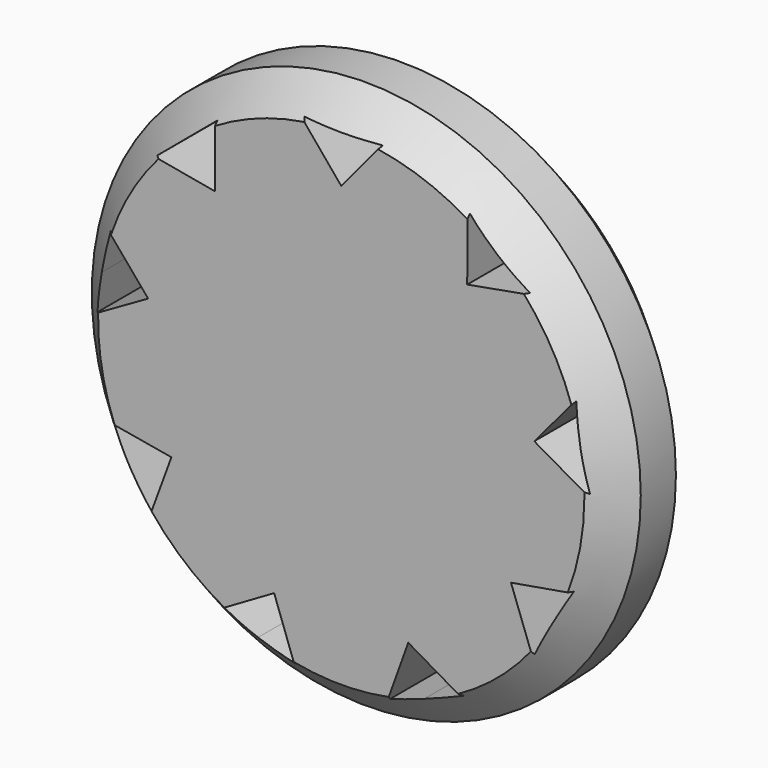
from build123d import *

# Parameters (mm, degrees)
F0_R     = 44.45
F1_DEPTH = 17.272
F3_DEPTH = 17.273


# Not quite as in the source:
# - a fillet or chamfer that OpenCascade refuses, or shapes differently, is made with other operations: its cross-section is extruded or revolved along the edge and cut away or added


with BuildPart() as f1:
    # F0 (on Front) → F1 (new body)
    with BuildSketch(Plane.XZ):
        Circle(F0_R)
    extrude(amount=F1_DEPTH)

    # F2 (on face) → F3 (cut, through all)
    with BuildSketch(Plane.XZ.offset(17.272)):
        Polygon((6.35, 39.37), (0, 39.37), (-6.35, 39.37), (0, 31.75), align=None)
        Polygon((-20.4085066075, 24.321911069), (-20.4421659796, 34.2408710471), (-25.3065481934, 30.1591697256), (-30.1709304072, 26.0774684041), align=None)
        Polygon((-31.2676461581, 5.5133296409), (-37.6692153079, 13.0900579864), (-38.7718812361, 6.8365287547), (-39.8745471643, 0.5829995231), align=None)
        Polygon((-27.4963065702, -15.875), (-37.270420147, -14.185738686), (-34.095420147, -19.685), (-30.920420147, -25.184261314), align=None)
        Polygon((-10.8591395506, -29.83524071), (-19.4323811847, -34.8238705702), (-13.4653330427, -36.9956984803), (-7.4982849007, -39.1675263905), align=None)
        Polygon((10.8591395506, -29.83524071), (7.4982849007, -39.1675263905), (13.4653330427, -36.9956984803), (19.4323811847, -34.8238705702), align=None)
        Polygon((27.4963065702, -15.875), (30.920420147, -25.184261314), (34.095420147, -19.685), (37.270420147, -14.185738686), align=None)
        Polygon((31.2676461581, 5.5133296409), (39.8745471643, 0.5829995231), (38.7718812361, 6.8365287547), (37.6692153079, 13.0900579864), align=None)
        Polygon((20.4085066075, 24.321911069), (30.1709304072, 26.0774684041), (25.3065481934, 30.1591697256), (20.4421659796, 34.2408710471), align=None)
    extrude(amount=-F3_DEPTH, mode=Mode.SUBTRACT)

    # F4: chamfer of 5.08 on 2 edges, made by hand

    # F4_s1 → F4_t2 (revolve, cut)
    with BuildSketch(Plane.XY):
        Polygon((44.45, -12.192), (39.37, -17.272), (44.45, -17.272), align=None)
    revolve(axis=Axis((0, -17.272, 0), (0, -1, 0)), mode=Mode.SUBTRACT)

    # F4_s3 → F4_t4 (revolve, cut)
    with BuildSketch(Plane.XY):
        Polygon((44.45, -5.08), (39.37, 0), (44.45, 0), align=None)
    revolve(axis=Axis((0, 0, 0), (0, -1, 0)), mode=Mode.SUBTRACT)


solid = f1.part
